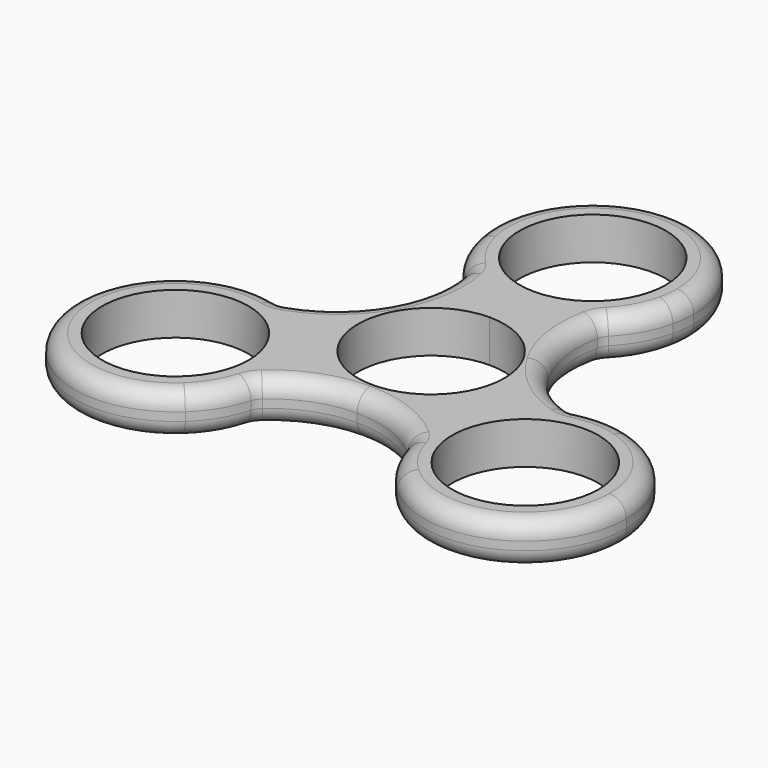
from build123d import *

# Parameters (mm, degrees)
F0_R     = 11.049
F1_DEPTH = 6.35
F2_R     = 2.54


with BuildPart() as f1:
    # F0 (on Top) → F1 (new body)
    with BuildSketch(Plane.XY):
        with BuildLine():
            ThreePointArc((0, 11.049), (7.8128228253, 7.8128228253), (11.049, 0))
            ThreePointArc((11.049, 0), (-2.8596916293, -10.6725144547), (-9.5687146864, 5.5245))
            Line((-9.5687146864, 5.5245), (-12.0983748909, 6.985))
            ThreePointArc((-12.0983748733, 6.9850000305), (-12.0983749042, -6.9849999769), (-1.8e-08, -13.97))
            ThreePointArc((-1.8e-08, -13.97), (9.8782817268, -9.8782817395), (13.97, 0))
            ThreePointArc((13.97, 0), (13.4939837796, 3.6157021111), (12.098374838, 6.9850000915))
            ThreePointArc((12.098374838, 6.9850000915), (6.9849999543, 12.0983749173), (0, 13.97))
            Line((0, 13.97), (0, 11.049))
        make_face()
        with BuildLine():
            ThreePointArc((-9.5687146864, 5.5245), (-5.5245, 9.5687146864), (0, 11.049))
            Line((0, 11.049), (0, 13.97))
            ThreePointArc((0, 13.97), (-6.9849999848, 12.0983748997), (-12.0983748733, 6.9850000305))
            Line((-12.0983748909, 6.985), (-9.5687146864, 5.5245))
        make_face()
        with BuildLine():
            Line((0, 15.24), (0, 13.97))
            ThreePointArc((0, 13.97), (6.9849999543, 12.0983749173), (12.098374838, 6.9850000915))
            ThreePointArc((12.098374838, 6.9850000915), (10.0392971957, 12.9986809188), (10.404817525, 19.3445892635))
            ThreePointArc((10.404817525, 19.3445892635), (5.5925817104, 16.3032362715), (0, 15.24))
        make_face()
        with BuildLine():
            ThreePointArc((-12.0983748733, 6.9850000305), (-6.9849999848, 12.0983748997), (0, 13.97))
            Line((0, 13.97), (0, 15.24))
            ThreePointArc((0, 15.24), (-5.5925817104, 16.3032362715), (-10.404817525, 19.3445892635))
            ThreePointArc((-10.404817525, 19.3445892635), (-10.0392972004, 12.9986808839), (-12.0983748733, 6.9850000305))
        make_face()
        with BuildLine():
            ThreePointArc((-1.8e-08, -13.97), (-12.0983749042, -6.9849999769), (-12.0983748733, 6.9850000305))
            ThreePointArc((-12.0983748733, 6.9850000305), (-16.2768364336, 2.1949459914), (-21.9553144904, -0.6614583333))
            ThreePointArc((-21.9553144904, -0.6614583333), (-14.1502187468, -6.1687644394), (-11.1564543073, -15.24))
            ThreePointArc((-11.1564543073, -15.24), (-11.2552854309, -16.9728026589), (-11.5504969654, -18.6831309301))
            ThreePointArc((-11.5504969654, -18.6831309301), (-6.237539253, -15.1936268504), (-1.8e-08, -13.97))
        make_face()
        with BuildLine():
            ThreePointArc((21.9553144904, -0.6614583333), (16.2768364057, 2.1949460129), (12.098374838, 6.9850000915))
            ThreePointArc((12.098374838, 6.9850000915), (13.4939837796, 3.6157021111), (13.97, 0))
            ThreePointArc((13.97, 0), (9.8782817268, -9.8782817395), (-1.8e-08, -13.97))
            ThreePointArc((-1.8e-08, -13.97), (6.2375392363, -15.1936268436), (11.5504969654, -18.6831309301))
            ThreePointArc((11.5504969654, -18.6831309301), (13.1982271537, -7.62), (21.9553144904, -0.6614583333))
        make_face()
        with BuildLine():
            ThreePointArc((-10.404817525, 19.3445892635), (-5.5925817104, 16.3032362715), (0, 15.24))
            ThreePointArc((0, 15.24), (5.5925817104, 16.3032362715), (10.404817525, 19.3445892635))
            ThreePointArc((10.404817525, 19.3445892635), (12.0983748909, 23.495), (14.8459573419, 27.0368690699))
            ThreePointArc((14.8459573419, 27.0368690699), (15.1411688765, 28.7471973411), (15.24, 30.48))
            ThreePointArc((15.24, 30.48), (-1.7328026589, 45.6211688765), (-14.8459573419, 27.0368690699))
            ThreePointArc((-14.8459573419, 27.0368690699), (-12.0983748909, 23.495), (-10.404817525, 19.3445892635))
        make_face()
        with BuildLine():
            ThreePointArc((11.049, 30.48), (7.8128228253, 22.6671771747), (0, 19.431))
            ThreePointArc((0, 19.431), (-7.8128228253, 38.2928228253), (11.049, 30.48))
        make_face(mode=Mode.SUBTRACT)
        with BuildLine():
            ThreePointArc((-30.8375941243, -0.6614583333), (-26.3964543073, -1.27), (-21.9553144904, -0.6614583333))
            ThreePointArc((-21.9553144904, -0.6614583333), (-26.3964543073, 0), (-30.8375941243, -0.6614583333))
        make_face()
        with BuildLine():
            ThreePointArc((-11.1564543073, -15.24), (-14.1502187468, -6.1687644394), (-21.9553144904, -0.6614583333))
            ThreePointArc((-21.9553144904, -0.6614583333), (-26.3964543073, -1.27), (-30.8375941243, -0.6614583333))
            ThreePointArc((-30.8375941243, -0.6614583333), (-39.594681461, -22.86), (-15.9916367823, -26.3754107365))
            ThreePointArc((-15.9916367823, -26.3754107365), (-14.2980794165, -22.225), (-11.5504969654, -18.6831309301))
            ThreePointArc((-11.5504969654, -18.6831309301), (-11.2552854309, -16.9728026589), (-11.1564543073, -15.24))
        make_face()
        with Locations((-26.3964543073, -15.24)):
            Circle(F0_R, mode=Mode.SUBTRACT)
        with BuildLine():
            ThreePointArc((-14.8459573419, 27.0368690699), (-13.1982271537, 22.86), (-10.404817525, 19.3445892635))
            ThreePointArc((-10.404817525, 19.3445892635), (-12.0983748909, 23.495), (-14.8459573419, 27.0368690699))
        make_face()
        with BuildLine():
            ThreePointArc((14.8459573419, 27.0368690699), (12.0983748909, 23.495), (10.404817525, 19.3445892635))
            ThreePointArc((10.404817525, 19.3445892635), (13.1982271537, 22.86), (14.8459573419, 27.0368690699))
        make_face()
        with BuildLine():
            ThreePointArc((30.8375941243, -0.6614583333), (26.3964543073, -1.27), (21.9553144904, -0.6614583333))
            ThreePointArc((21.9553144904, -0.6614583333), (13.1982271537, -7.62), (11.5504969654, -18.6831309301))
            ThreePointArc((11.5504969654, -18.6831309301), (14.2980794165, -22.225), (15.9916367823, -26.3754107365))
            ThreePointArc((15.9916367823, -26.3754107365), (32.4663876232, -29.2190382194), (41.6364543073, -15.24))
            ThreePointArc((41.6364543073, -15.24), (38.6426898679, -6.1687644394), (30.8375941243, -0.6614583333))
        make_face()
        with Locations((26.3964543073, -15.24)):
            Circle(F0_R, mode=Mode.SUBTRACT)
        with BuildLine():
            ThreePointArc((30.8375941243, -0.6614583333), (26.3964543073, 0), (21.9553144904, -0.6614583333))
            ThreePointArc((21.9553144904, -0.6614583333), (26.3964543073, -1.27), (30.8375941243, -0.6614583333))
        make_face()
        with BuildLine():
            ThreePointArc((15.9916367823, -26.3754107365), (14.2980794165, -22.225), (11.5504969654, -18.6831309301))
            ThreePointArc((11.5504969654, -18.6831309301), (13.1982271537, -22.86), (15.9916367823, -26.3754107365))
        make_face()
        with BuildLine():
            ThreePointArc((-15.9916367823, -26.3754107365), (-13.1982271537, -22.86), (-11.5504969654, -18.6831309301))
            ThreePointArc((-11.5504969654, -18.6831309301), (-14.2980794165, -22.225), (-15.9916367823, -26.3754107365))
        make_face()
    extrude(amount=F1_DEPTH)

    # F2
    f2_edges = [f1.edges().sort_by_distance(p)[0] for p in [
        (-12.098375, 6.985, 6.35),
        (0, 45.72, 6.35),
        (12.098375, 6.985, 6.35),
        (39.594681, -22.86, 6.35),
        (0, -13.97, 6.35),
        (-39.594681, -22.86, 6.35),
        (-39.594681, -22.86, 0),
        (-21.955314, -0.661458, 3.175),
        (-11.550497, -18.683131, 3.175),
        (10.404818, 19.344589, 3.175),
        (-10.404818, 19.344589, 3.175),
        (0, 45.72, 0),
        (11.550497, -18.683131, 3.175),
        (0, -13.97, 0),
        (21.955314, -0.661458, 3.175),
        (39.594681, -22.86, 0),
        (-12.098375, 6.985, 0),
        (12.098375, 6.985, 0),
    ]]
    fillet(f2_edges, radius=F2_R)


solid = f1.part
